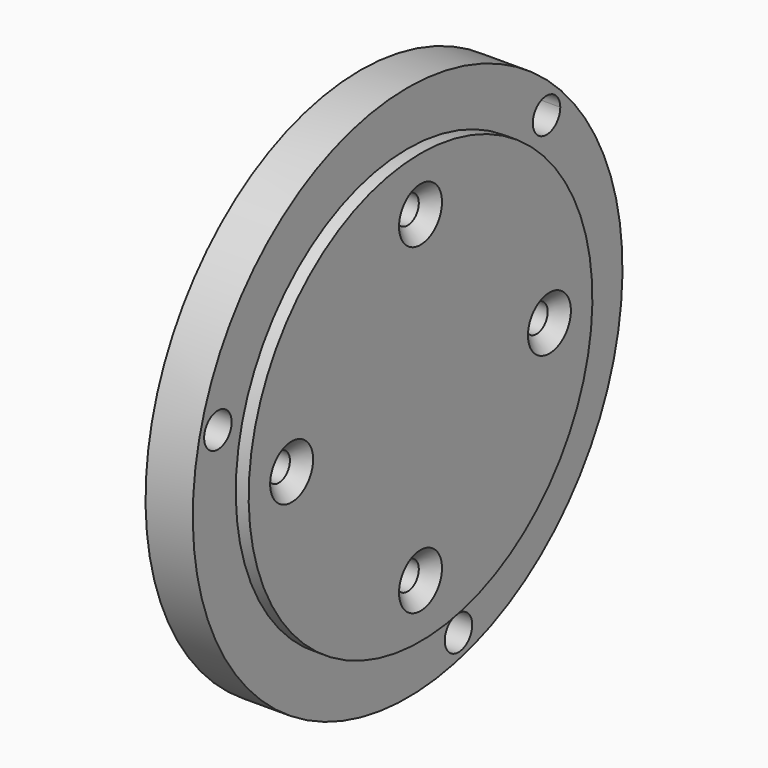
from build123d import *

# Parameters (mm, degrees)
F2_R     = 4
F3_DEPTH = 25
F4_R     = 3.25
F5_DEPTH = 25
F6_SIZE  = 3


# Not quite as in the source:
# - a feature names something its author has since deleted; it is built from what else it names


with BuildPart() as f1:
    # F0 (on Front) → F1 (revolve)
    with BuildSketch(Plane.XZ):
        Polygon((0, 9.55), (0, 0), (17.623, 0), (24, 0), (24, 50), (21, 50), (21, 62.5), (10, 62.5), (10, 50.8), (4, 50.8), (4, 9.55), align=None)
    revolve(axis=Axis((8.8115, 0, 0), (1, 0, 0)))

    # F2 (on face) → F3 (cut)
    with BuildSketch(Plane.YZ.offset(21)):
        with BuildLine():
            ThreePointArc((44.4111525448, 40.4111525448), (38.8804188154, 44.1066706749), (37.5827254201, 37.5827254201))
            ThreePointArc((37.5827254201, 37.5827254201), (41.9418862743, 36.7156344148), (44.4111525448, 40.4111525448))
        make_face()
        with Locations((-55.2026609724, 14.7915084276)):
            Circle(F2_R)
        with Locations((14.7915084276, -55.2026609724)):
            Circle(F2_R)
    extrude(amount=-F3_DEPTH, mode=Mode.SUBTRACT)

    # F4 (on face) → F5 (cut)
    with BuildSketch(Plane(origin=(4, 0, 0), x_dir=(0, -1, 0), z_dir=(-1, 0, 0))):
        with Locations((0, 37.5)):
            Circle(F4_R)
        with Locations((-37.5, 0)):
            Circle(F4_R)
        with Locations((0, -37.5)):
            Circle(F4_R)
        with Locations((37.5, 0)):
            Circle(F4_R)
    extrude(amount=-F5_DEPTH, mode=Mode.SUBTRACT)

    # F6
    f6_edges = [f1.edges().sort_by_distance(p)[0] for p in [
        (24, -34.25, 0),
        (24, 3.25, 37.5),
        (24, 40.75, 0),
        (24, 3.25, -37.5),
    ]]
    chamfer(f6_edges, length=F6_SIZE)


solid = f1.part
